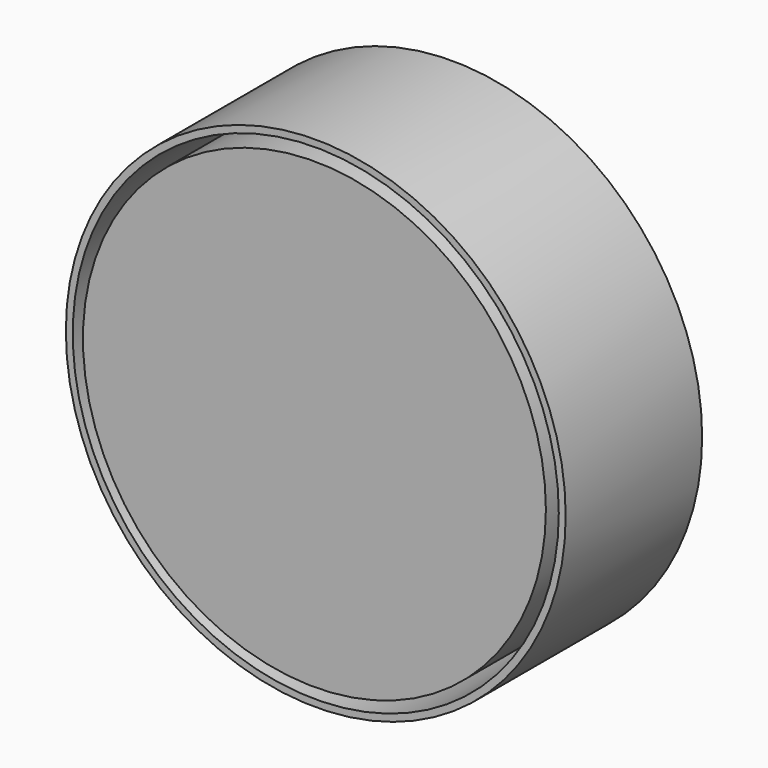
from build123d import *

# Parameters (mm, degrees)
F0_R     = 17.0643351891
F1_DEPTH = 12.7
F5_R     = 18.4248242349
F6_DEPTH = 12.5755444169
F7_T     = -0.508


# Not quite as in the source:
# - the program builds the solid bodies; features that only make, move or delete a surface that nothing else refers to are left out


with BuildPart() as f1:
    # F0 (on Front) → F1 (new body)
    with BuildSketch(Plane.XZ):
        Circle(F0_R)
    extrude(amount=F1_DEPTH)


with BuildPart() as f6:
    # F5 (on Front) → F6 (new body)
    with BuildSketch(Plane.XZ):
        Circle(F5_R)
    extrude(amount=F6_DEPTH)

    # F7
    f7_openings = [f6.faces().sort_by_distance(p)[0] for p in [
        (0, -12.575544, 0),
    ]]
    offset(amount=F7_T, openings=f7_openings)


solid = Compound([f1.part, f6.part])
